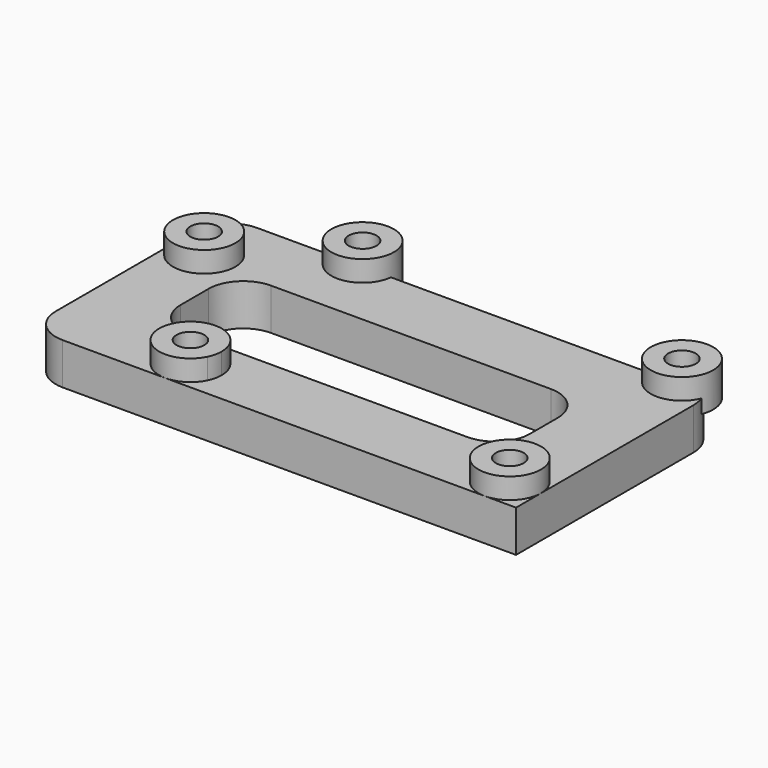
from build123d import *

# Parameters (mm, degrees)
F4_R          = 4.5
F4_R_2        = 2
F5_DEPTH      = 9
F6_W          = 70.3
F6_H          = 35.0108387947
F6_W_2        = 50.3
F6_H_2        = 15.0108387947
F7_DEPTH      = 6
F8_R          = 4.5
F8_R_2        = 2
F9_DEPTH      = 5
F10_R         = 2
F11_DEPTH     = 9.001
F13_START     = -5
F12_R         = 3.5
F12_R_2       = 2
F13_DEPTH     = 23
F14_R         = 2
F15_DEPTH     = 9.001
F16_T1_DEPTH  = 6
F16_T3_DEPTH  = 6
F16_T5_DEPTH  = 6
F16_T7_DEPTH  = 6
F16_T9_DEPTH  = 31
F16_T14_DEPTH = 21.2263176167
F16_T19_DEPTH = 21.2263176167
F16_S20_R     = 4.5
F16_T21_DEPTH = 12
F16_T22_DEPTH = 31


# Not quite as in the source:
# - a fillet or chamfer that OpenCascade refuses, or shapes differently, is made with other operations: its cross-section is extruded or revolved along the edge and cut away or added
# - after a boolean that leaves OpenCascade's solid faulty, fix() repairs it


with BuildPart() as f5:
    # F4 (on Top) → F5 (new body)
    with BuildSketch(Plane.XY):
        with Locations((-30.4, 10.8)):
            Circle(F4_R)
        with Locations((-30.4, 10.8)):
            Circle(F4_R_2, mode=Mode.SUBTRACT)
    extrude(amount=F5_DEPTH)



with BuildPart() as f5b:
    # F4 (on Top) → F5, piece 2 (new body)
    with BuildSketch(Plane.XY):
        with Locations((30.9, -10.8)):
            Circle(F4_R)
        with Locations((30.9, -10.8)):
            Circle(F4_R_2, mode=Mode.SUBTRACT)
    extrude(amount=F5_DEPTH)


with BuildPart() as f5_1:
    add(f5.part)

    add(f5b.part)  # F7 merges F5b
    # F6 (on face) → F7 (join)
    with BuildSketch(Plane.XY):
        with Locations((0.25, 2.2054193974)):
            Rectangle(F6_W, F6_H)
        with Locations((0.25, 2.2054193974)):
            Rectangle(F6_W_2, F6_H_2, mode=Mode.SUBTRACT)
    extrude(amount=F7_DEPTH)

    # F8 (on face) → F9 (join)
    with BuildSketch(Plane.XY.offset(9)):
        with BuildLine():
            Line((-19.1311288741, -12.8), (-15.1, -12.8))
            Line((-15.1, -12.8), (-11.0688711259, -12.8))
            ThreePointArc((-11.0688711259, -12.8), (-10.7187855603, -11.8271124735), (-10.6, -10.8))
            ThreePointArc((-10.6, -10.8), (-16.1271124735, -6.4187855603), (-19.1311288741, -12.8))
        make_face()
        with BuildLine():
            ThreePointArc((-15.1, -12.8), (-16.5142135624, -9.3857864376), (-13.1, -10.8))
            ThreePointArc((-13.1, -10.8), (-13.6857864376, -12.2142135624), (-15.1, -12.8))
        make_face(mode=Mode.SUBTRACT)
        with BuildLine():
            Line((-11.0688711259, -12.8), (-15.1, -12.8))
            Line((-15.1, -12.8), (-19.1311288741, -12.8))
            ThreePointArc((-19.1311288741, -12.8), (-15.1, -15.3), (-11.0688711259, -12.8))
        make_face()
        with Locations((-15.1, 20.2)):
            Circle(F8_R)
        with Locations((-15.1, 20.2)):
            Circle(F8_R_2, mode=Mode.SUBTRACT)
        with Locations((30.9, 20.2)):
            Circle(F8_R)
        with Locations((30.9, 20.2)):
            Circle(F8_R_2, mode=Mode.SUBTRACT)
    extrude(amount=-F9_DEPTH)

    # F10 (on face) → F11 (cut, through all)
    with BuildSketch(Plane.XY.offset(9)):
        with Locations((30.9, -10.8)):
            Circle(F10_R)
        with Locations((-30.4, 10.8)):
            Circle(F10_R)
    extrude(amount=-F11_DEPTH, mode=Mode.SUBTRACT)

    # F12 (on face) → F13 (cut)
    with BuildSketch(Plane.XY.offset(9).offset(F13_START)):
        with Locations((-15.1, 20.2)):
            Circle(F12_R)
        with Locations((-15.1, 20.2)):
            Circle(F12_R_2, mode=Mode.SUBTRACT)
        with Locations((30.9, 20.2)):
            Circle(F12_R)
        with Locations((30.9, 20.2)):
            Circle(F12_R_2, mode=Mode.SUBTRACT)
        with Locations((-15.1, -10.8)):
            Circle(F12_R)
        with Locations((-15.1, -10.8)):
            Circle(F12_R_2, mode=Mode.SUBTRACT)
    extrude(amount=-F13_DEPTH, mode=Mode.SUBTRACT)

    # F14 (on face) → F15 (cut, through all)
    with BuildSketch(Plane.XY.offset(9)):
        with Locations((-15.1, 20.2)):
            Circle(F14_R)
        with Locations((30.9, 20.2)):
            Circle(F14_R)
        with Locations((-15.1, -10.8)):
            Circle(F14_R)
        with Locations((30.9, -10.8)):
            Circle(F14_R)
    extrude(amount=-F15_DEPTH, mode=Mode.SUBTRACT)

    add(f5_1.part.fix(), mode=Mode.REPLACE)

    # F16: fillet of radius 5 on 7 edges, made by hand

    # F16_s2 → F16_t1 (join)
    with BuildSketch(Plane.XY):
        with BuildLine():
            ThreePointArc((-24.9, -0.3), (-23.4355339059, -3.8355339059), (-19.9, -5.3))
            Line((-19.9, -5.3), (-24.9, -5.3))
            Line((-24.9, -5.3), (-24.9, -0.3))
        make_face()
    extrude(amount=F16_T1_DEPTH)

    # F16_s4 → F16_t3 (join)
    with BuildSketch(Plane.XY):
        with BuildLine():
            ThreePointArc((-24.9, 4.7108387947), (-23.4355339059, 8.2463727006), (-19.9, 9.7108387947))
            Line((-19.9, 9.7108387947), (-24.9, 9.7108387947))
            Line((-24.9, 9.7108387947), (-24.9, 4.7108387947))
        make_face()
    extrude(amount=F16_T3_DEPTH)

    # F16_s6 → F16_t5 (join)
    with BuildSketch(Plane.XY):
        with BuildLine():
            ThreePointArc((25.4, -0.3), (23.9355339059, -3.8355339059), (20.4, -5.3))
            Line((20.4, -5.3), (25.4, -5.3))
            Line((25.4, -5.3), (25.4, -0.3))
        make_face()
    extrude(amount=F16_T5_DEPTH)

    # F16_s8 → F16_t7 (join)
    with BuildSketch(Plane.XY):
        with BuildLine():
            ThreePointArc((25.4, 4.7108387947), (23.9355339059, 8.2463727006), (20.4, 9.7108387947))
            Line((20.4, 9.7108387947), (25.4, 9.7108387947))
            Line((25.4, 9.7108387947), (25.4, 4.7108387947))
        make_face()
    extrude(amount=F16_T7_DEPTH)

    # F16_s10 → F16_t9 (cut)
    with BuildSketch(Plane.XY.offset(-12.5)):
        with BuildLine():
            ThreePointArc((-34.9, -10.3), (-33.4355339059, -13.8355339059), (-29.9, -15.3))
            Line((-29.9, -15.3), (-34.9, -15.3))
            Line((-34.9, -15.3), (-34.9, -10.3))
        make_face()
    extrude(amount=F16_T9_DEPTH, mode=Mode.SUBTRACT)


with BuildPart() as f16_tool12:
    # F16_s13 → F16_t14 (new body)
    with BuildSketch(Plane.XY.offset(-7.6131588083)):
        with BuildLine():
            ThreePointArc((34.3656487582, 19.7108387947), (35.1343554889, 18.2736418448), (35.4, 16.6655752714))
            Line((35.4, 16.6655752714), (35.4, 19.7108387947))
            Line((35.4, 19.7108387947), (34.3656487582, 19.7108387947))
        make_face()
    extrude(amount=F16_T14_DEPTH)

    split(bisect_by=Plane.XY.offset(4), keep=Keep.BOTTOM)


with BuildPart() as f5_2:
    add(f5_1.part)

    # F16_t11: cut F16_tool12
    add(f16_tool12.part, mode=Mode.SUBTRACT)


with BuildPart() as f16_tool17:
    # F16_s18 → F16_t19 (new body)
    with BuildSketch(Plane.XY.offset(-7.6131588083)):
        with BuildLine():
            ThreePointArc((34.3656487582, 19.7108387947), (35.1343554889, 18.2736418448), (35.4, 16.6655752714))
            Line((35.4, 16.6655752714), (35.4, 19.7108387947))
            Line((35.4, 19.7108387947), (34.3656487582, 19.7108387947))
        make_face()
    extrude(amount=F16_T19_DEPTH)

    # F16_s20 → F16_t21 (cut, symmetric)
    with BuildSketch(Plane.XY.offset(3)):
        with Locations((30.9, 20.2)):
            Circle(F16_S20_R)
    extrude(amount=F16_T21_DEPTH, both=True, mode=Mode.SUBTRACT)


with BuildPart() as f5_3:
    add(f5_2.part)

    # F16_t16: cut F16_tool17
    add(f16_tool17.part, mode=Mode.SUBTRACT)

    # F16_s23 → F16_t22 (cut)
    with BuildSketch(Plane.XY.offset(-12.5)):
        with BuildLine():
            ThreePointArc((-29.9, 19.7108387947), (-33.4355339059, 18.2463727006), (-34.9, 14.7108387947))
            Line((-34.9, 14.7108387947), (-34.9, 19.7108387947))
            Line((-34.9, 19.7108387947), (-29.9, 19.7108387947))
        make_face()
    extrude(amount=F16_T22_DEPTH, mode=Mode.SUBTRACT)


solid = f5_3.part
